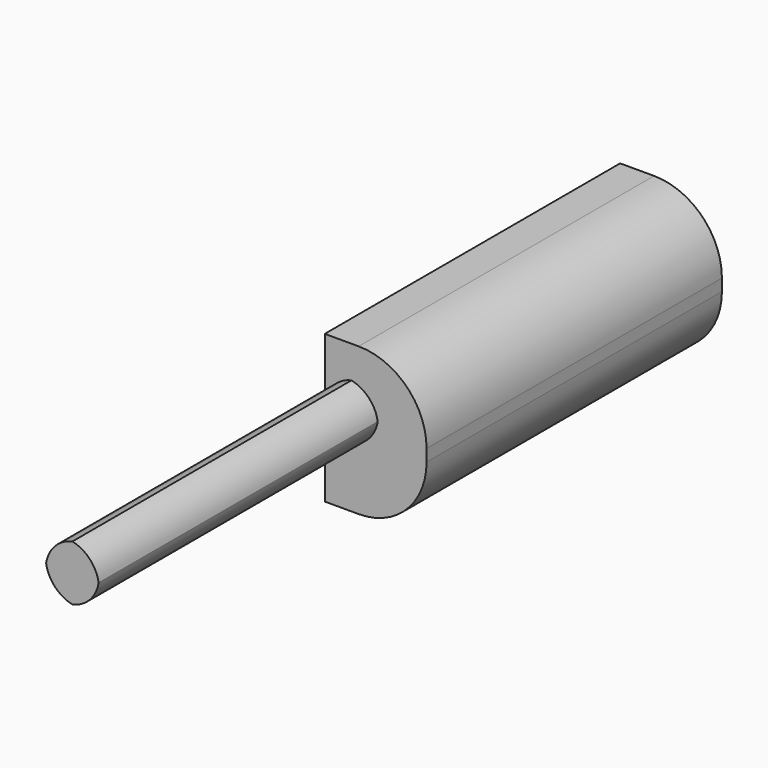
from build123d import *

# Parameters (mm, degrees)
F0_W        = 39.7763997316
F0_H        = 4.2672008276
F1_DEPTH    = 4
F2_T1_DEPTH = 52.4763997316
F3_W        = 27.6340441778
F3_H        = 11.0536180437
F4_DEPTH    = 7.62
F5_R        = 5.08
F6_R        = 1.45
F7_DEPTH    = 3.81


# Not quite as in the source:
# - a fillet or chamfer that OpenCascade refuses, or shapes differently, is made with other operations: its cross-section is extruded or revolved along the edge and cut away or added


with BuildPart() as f1:
    # F0 (on Right) → F1 (new body)
    with BuildSketch(Plane.YZ):
        with Locations((-19.8881998658, 24.0791998804)):
            Rectangle(F0_W, F0_H)
    extrude(amount=F1_DEPTH)

    # F2: fillet of radius 2.54 on 4 edges, made by hand

    # F2_s2 → F2_t1 (cut)
    with BuildSketch(Plane.XZ.offset(-6.35)):
        with BuildLine():
            ThreePointArc((1.46, 26.2128002942), (3.2560512242, 25.4688515184), (4, 23.6728002942))
            Line((4, 23.6728002942), (4, 26.2128002942))
            Line((4, 26.2128002942), (1.46, 26.2128002942))
        make_face()
        with BuildLine():
            ThreePointArc((2.54, 26.2128002942), (0.7439487758, 25.4688515184), (0, 23.6728002942))
            Line((0, 23.6728002942), (0, 26.2128002942))
            Line((0, 26.2128002942), (2.54, 26.2128002942))
        make_face()
        with BuildLine():
            ThreePointArc((1.46, 21.9455994666), (3.2560512242, 22.6895482423), (4, 24.4855994666))
            Line((4, 24.4855994666), (4, 21.9455994666))
            Line((4, 21.9455994666), (1.46, 21.9455994666))
        make_face()
        with BuildLine():
            ThreePointArc((2.54, 21.9455994666), (0.7439487758, 22.6895482423), (0, 24.4855994666))
            Line((0, 24.4855994666), (0, 21.9455994666))
            Line((0, 21.9455994666), (2.54, 21.9455994666))
        make_face()
    extrude(amount=F2_T1_DEPTH, mode=Mode.SUBTRACT)

    # F3 (on Right) → F4 (join)
    with BuildSketch(Plane.YZ):
        with Locations((0.1553441398, 23.0435747653)):
            Rectangle(F3_W, F3_H)
    extrude(amount=F4_DEPTH)

    # F5
    f5_edges = [f1.edges().sort_by_distance(p)[0] for p in [
        (7.62, 0.155344, 28.570384),
        (7.62, 0.155344, 17.516766),
    ]]
    fillet(f5_edges, radius=F5_R)

    # F6 (on face) → F7 (join)
    with BuildSketch(Plane(origin=(0, 0, 0), x_dir=(0, -1, 0), z_dir=(-1, 0, 0))):
        with Locations((0, 22.1642478059)):
            Circle(F6_R)
    extrude(amount=F7_DEPTH)


solid = f1.part
